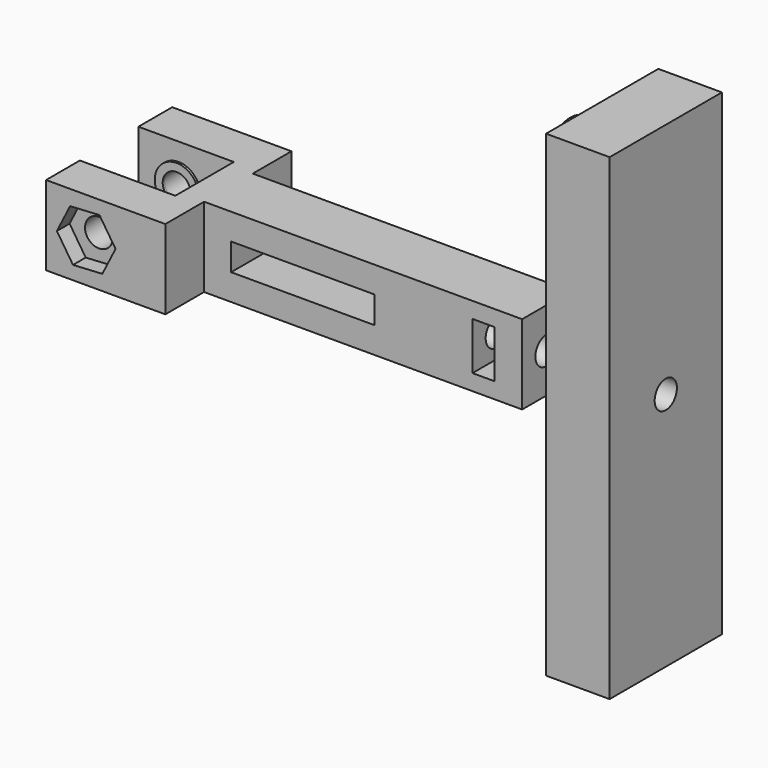
from build123d import *

# Parameters (mm, degrees)
F0_W      = 40
F0_H      = 3.825
F1_DEPTH  = 10
F2_R      = 1.75
F3_DEPTH  = 19.8241538475
F4_W      = 18
F4_H      = 3.4
F4_W_2    = 2.75
F4_H_2    = 6
F5_DEPTH  = 13.7375769237
F6_R      = 1.75
F7_DEPTH  = 15
F10_DEPTH = 2
F11_W     = 17.65
F11_H     = 60
F12_DEPTH = 8
F13_R     = 1.75
F14_DEPTH = 70.001
F15_R     = 2.75
F15_R_2   = 1.75
F16_DEPTH = 0.3
F17_R     = 1.75
F18_DEPTH = 2
F19_R     = 3.75
F20_DEPTH = 4


# Not quite as in the source:
# - a pattern or mirror of a feature is missing from the dataset's text; its kind, count and spacing are read off the source's solid


with BuildPart() as f1:
    # F0 (on Top) → F1 (new body)
    with BuildSketch(Plane.XY):
        Polygon((0, -3.825), (0, 0), (-3, 0), (-3, -4.6), (-15, -4.6), (-15, -9.9115769237), (0, -9.9115769237), align=None)
        Polygon((-3, 0), (0, 0), (0, 3.825), (0, 9.9115769237), (-15, 9.9115769237), (-15, 4.6), (-3, 4.6), align=None)
        with Locations((20, 1.9125)):
            Rectangle(F0_W, F0_H)
        with Locations((20, -1.9125)):
            Rectangle(F0_W, F0_H)
    extrude(amount=F1_DEPTH)

    # F2 (on face) → F3 (cut, through all)
    with BuildSketch(Plane.XZ.offset(9.9115769237)):
        with Locations((-9.9527407438, 5)):
            Circle(F2_R)
    extrude(amount=-F3_DEPTH, mode=Mode.SUBTRACT)

    # F4 (on face) → F5 (cut, through all)
    with BuildSketch(Plane.XZ.offset(3.825)):
        with Locations((12.4002694301, 5)):
            Rectangle(F4_W, F4_H)
        with Locations((35.125, 5)):
            Rectangle(F4_W_2, F4_H_2)
    extrude(amount=-F5_DEPTH, mode=Mode.SUBTRACT)

    # F6 (on face) → F7 (cut)
    with BuildSketch(Plane.YZ.offset(40)):
        with Locations((0, 5)):
            Circle(F6_R)
    extrude(amount=-F7_DEPTH, mode=Mode.SUBTRACT)

    # F15 (on face) → F16 (join)
    with BuildSketch(Plane.XZ.offset(-4.6)):
        with Locations((-9.9527407438, 5)):
            Circle(F15_R)
        with Locations((-9.9527407438, 5)):
            Circle(F15_R_2, mode=Mode.SUBTRACT)
    f16 = extrude(amount=F16_DEPTH)

    # F16_copies: F16 across plane
    add(f16.mirror(Plane(origin=(0, 0, 0), x_dir=(0, 0, -1), z_dir=(0, -1, 0))))

    # F17 (on face) → F18 (cut)
    with BuildSketch(Plane.XZ.offset(9.9115769237)):
        Polygon((-7.9284293953, 1.9088033227), (-6.2635302189, 5.2075067143), (-8.2878415673, 8.2987033916), (-11.9770520922, 8.0911966773), (-13.6419512686, 4.7924932857), (-11.6176399202, 1.7012966084), align=None)
        with Locations((-9.9527407438, 5)):
            Circle(F17_R, mode=Mode.SUBTRACT)
    f18 = extrude(amount=-F18_DEPTH, mode=Mode.SUBTRACT)

    # F18_copies: F18 across plane
    add(f18.mirror(Plane.ZX), mode=Mode.SUBTRACT)


with BuildPart() as f10:
    # F9 (on offset) → F10 (new body)
    with BuildSketch(Plane.YZ.offset(45)):
        Polygon((3.825, 0), (3.825, 10), (3.825, 19.8484882712), (-3.825, 19.8484882712), (-3.825, 10), (-3.825, 0), (-3.825, -10.1515117288), (3.825, -10.1515117288), align=None)
    extrude(amount=F10_DEPTH)

    # F11 (on face) → F12 (join)
    with BuildSketch(Plane.YZ.offset(47)):
        with Locations((0, 4.8484882712)):
            Rectangle(F11_W, F11_H)
    extrude(amount=F12_DEPTH)

    # F13 (on face) → F14 (cut, through all)
    with BuildSketch(Plane.YZ.offset(55)):
        with Locations((0, 5)):
            Circle(F13_R)
    extrude(amount=-F14_DEPTH, mode=Mode.SUBTRACT)

    # F19 (on face) → F20 (join)
    with BuildSketch(Plane(origin=(47, 0, 0), x_dir=(0, -1, 0), z_dir=(-1, 0, 0))):
        with Locations((0, 28)):
            Circle(F19_R)
        with Locations((0, -18)):
            Circle(F19_R)
    extrude(amount=F20_DEPTH)


solid = Compound([f1.part, f10.part])
